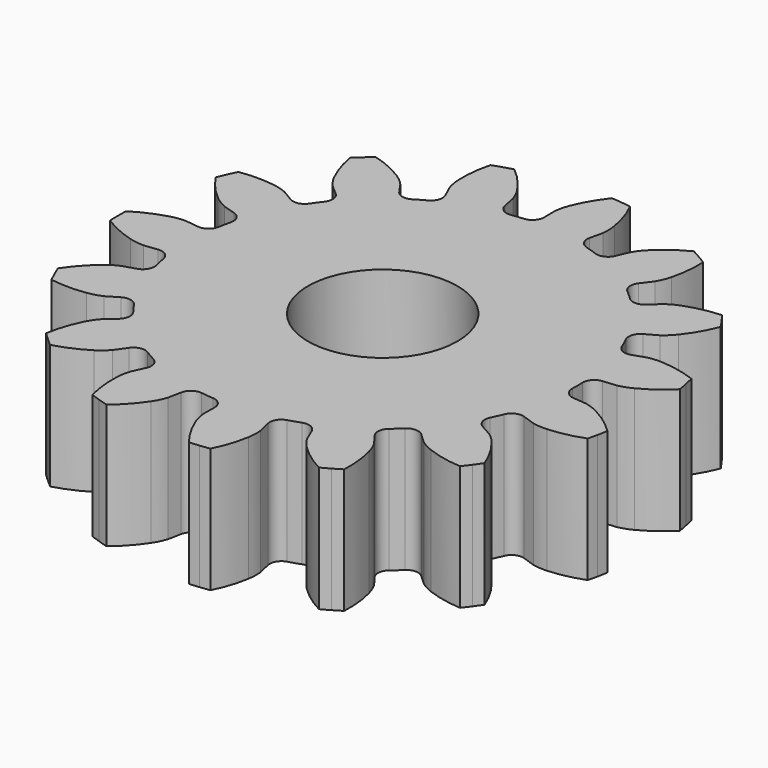
from build123d import *

# Parameters (mm, degrees)
F1_R            = 7.8125
F2_DEPTH        = 5
F4_DEPTH        = 5
F4_COPIES_COUNT = 15
F5_R            = 3
F6_DEPTH        = 3.5
F7_R            = 1.5
F8_DEPTH        = 1.501


# Not quite as in the source:
# - a pattern or mirror of a feature is missing from the dataset's text; its kind, count and spacing are read off the source's solid


with BuildPart() as f2:
    # F1 (on Top) → F2 (new body)
    with BuildSketch(Plane.XY):
        Circle(F1_R)
    extrude(amount=F2_DEPTH)

    # F3 (on Top) → F4 (join)
    with BuildSketch(Plane.XY):
        with BuildLine():
            ThreePointArc((1.1126473792, 10.5665813208), (0.9137266594, 10.5856378453), (0.7144827287, 10.6009499306))
            ThreePointArc((0.7144827287, 10.6009499306), (0.3106908097, 10.0151045947), (0, 9.375))
            ThreePointArc((0, 9.375), (0.9817476875, 9.3234541066), (1.9526996285, 9.1693832487))
            ThreePointArc((1.9526996285, 9.1693832487), (1.782149111, 9.8601619342), (1.5092378696, 10.5172632397))
            ThreePointArc((1.5092378696, 10.5172632397), (1.3111745241, 10.543787098), (1.1126473792, 10.5665813208))
        make_face()
        with BuildLine():
            ThreePointArc((1.9526996285, 9.1693832487), (0.9817476875, 9.3234541066), (0, 9.375))
            ThreePointArc((0, 9.375), (-0.088963902, 9.0964356851), (-0.1400392587, 8.8085052051))
            Line((-0.1400392587, 8.8085052051), (-0.1314291659, 8.2669281704))
            ThreePointArc((-0.1314291659, 8.2669281704), (-0.2543373669, 7.9429946483), (-0.5661508852, 7.7919592803))
            ThreePointArc((-0.5661508852, 7.7919592803), (0.8181230729, 7.7695450888), (2.1767051131, 7.5031400827))
            ThreePointArc((2.1767051131, 7.5031400827), (1.903189279, 7.7158098763), (1.8504482091, 8.05823904))
            Line((1.8504482091, 8.05823904), (1.9716734372, 8.5861445829))
            ThreePointArc((1.9716734372, 8.5861445829), (1.9816907409, 8.8783984229), (1.9526996285, 9.1693832487))
        make_face()
    f4 = extrude(amount=F4_DEPTH)

    # F4_copies: F4 ×15 about axis
    f4_copies_axis = Axis((0, 0, 0), (0, 0, 1))
    for i in range(1, F4_COPIES_COUNT):
        add(f4.rotate(f4_copies_axis, i * 360 / F4_COPIES_COUNT))

    # F5 (on face) → F6 (cut)
    with BuildSketch(Plane.XY.offset(5)):
        Circle(F5_R)
    extrude(amount=-F6_DEPTH, mode=Mode.SUBTRACT)

    # F7 (on face) → F8 (cut, through all)
    with BuildSketch(Plane.XY.offset(1.5)):
        Circle(F7_R)
    extrude(amount=-F8_DEPTH, mode=Mode.SUBTRACT)


solid = f2.part
